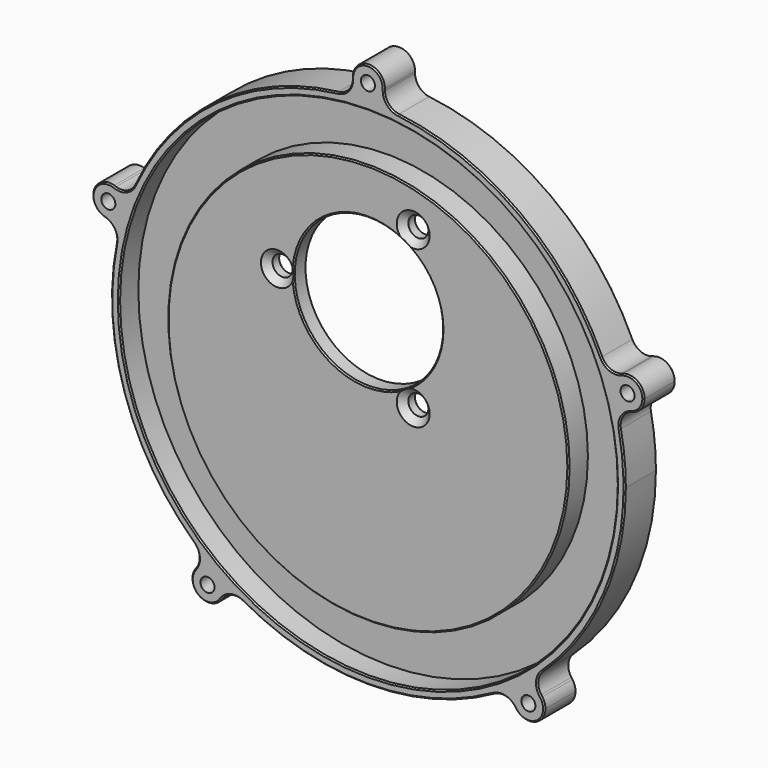
from build123d import *

# Parameters (mm, degrees)
F0_R          = 2.778125
F0_R_2        = 98.425
F1_DEPTH      = 15.875
F0_R_3        = 79.375
F0_R_4        = 3.96875
F0_R_5        = 29.36875
F2_DEPTH      = 6.35
F3_R          = 76.2
F3_R_2        = 3.96875
F3_R_3        = 29.36875
F4_DEPTH      = 9.525
F5_R          = 6.35
F7_T1_DEPTH   = 0.7496618475
F7_T3_DEPTH   = 0.7496618475
F7_T5_DEPTH   = 0.7496618475
F7_T7_DEPTH   = 0.7496618475
F7_T9_DEPTH   = 0.7496618475
F7_T11_DEPTH  = 0.7496618475
F7_T13_DEPTH  = 0.7496618475
F7_T15_DEPTH  = 0.7496618475
F7_T17_DEPTH  = 0.7496618475
F7_T20_ANGLE  = 58.4873459388
F7_T26_ANGLE  = 60.8393567081
F7_T28_ANGLE  = 121.6812910479
F7_T30_ANGLE  = 121.6812910479
F7_T32_ANGLE  = 60.8393567081
F7_T38_ANGLE  = 58.4873459388
F7_T46_ANGLE  = 83.2436729694
F7_T48_ANGLE  = 83.2436729694
F7_T50_ANGLE  = 180
F7_T52_ANGLE  = 83.2436729694
F7_T54_ANGLE  = 58.4873459388
F7_T56_ANGLE  = 83.2436729694
F7_T58_ANGLE  = 180
F7_T60_ANGLE  = 83.2436729694
F7_T62_ANGLE  = 58.4873459388
F7_T64_ANGLE  = 83.2436729694
F7_T66_ANGLE  = 180
F7_T68_ANGLE  = 83.2436729694
F7_T70_ANGLE  = 58.4873459388
F7_T72_ANGLE  = 83.2436729694
F7_T74_ANGLE  = 180
F7_T76_ANGLE  = 83.2436729694
F7_T78_ANGLE  = 58.4873459388
F7_T80_ANGLE  = 83.2436729694
F7_T82_ANGLE  = 180
F7_T84_ANGLE  = 83.2436729694
F7_T86_ANGLE  = 83.2436729694
F7_T88_ANGLE  = 180
F7_T90_ANGLE  = 83.2436729694
F7_T92_ANGLE  = 58.4873459388
F7_T94_ANGLE  = 83.2436729694
F7_T96_ANGLE  = 180
F7_T98_ANGLE  = 83.2436729694
F7_T100_ANGLE = 58.4873459388
F7_T102_ANGLE = 83.2436729694
F7_T104_ANGLE = 180
F7_T106_ANGLE = 83.2436729694
F7_T108_ANGLE = 58.4873459388
F7_T110_ANGLE = 83.2436729694
F7_T112_ANGLE = 180
F7_T114_ANGLE = 83.2436729694
F7_T116_ANGLE = 58.4873459388
F7_T118_ANGLE = 83.2436729694
F7_T120_ANGLE = 180


# Not quite as in the source:
# - a fillet or chamfer that OpenCascade refuses, or shapes differently, is made with other operations: its cross-section is extruded or revolved along the edge and cut away or added


with BuildPart() as f1:
    # F0 (on Front) → F1 (new body)
    with BuildSketch(Plane.XZ):
        with BuildLine():
            Line((-58.3141600707, -91.0658208948), (-54.4649709547, -85.7678665871))
            ThreePointArc((-54.4649709547, -85.7678665871), (-57.1199008944, -84.0230737465), (-59.7189814526, -82.1961267595))
            ThreePointArc((-59.7189814526, -82.1961267595), (-57.7935265058, -84.4505449687), (-57.101417985, -87.3333845428))
            ThreePointArc((-57.101417985, -87.3333845428), (-57.4122091065, -89.2956424571), (-58.3141600707, -91.0658208948))
        make_face()
        with BuildLine():
            ThreePointArc((-68.5886758993, -83.6009481907), (-64.4447767279, -81.0615635626), (-59.7189814526, -82.1961267595))
            ThreePointArc((-59.7189814526, -82.1961267595), (-62.2596715362, -80.2888117996), (-64.7394867833, -78.302993883))
            Line((-64.7394867833, -78.302993883), (-68.5886758993, -83.6009481907))
        make_face()
        with BuildLine():
            ThreePointArc((-57.101417985, -87.3333845428), (-57.7935265058, -84.4505449687), (-59.7189814526, -82.1961267595))
            ThreePointArc((-59.7189814526, -82.1961267595), (-64.4447767279, -81.0615635626), (-68.5886758993, -83.6009481907))
            ThreePointArc((-68.5886758993, -83.6009481907), (-67.183854337, -92.4706424571), (-58.3141600707, -91.0658208948))
            ThreePointArc((-58.3141600707, -91.0658208948), (-57.4122091065, -89.2956424571), (-57.101417985, -87.3333845428))
        make_face()
        with Locations((-63.451417985, -87.3333845428)):
            Circle(F0_R, mode=Mode.SUBTRACT)
        with BuildLine():
            Line((68.5886758993, -83.6009481907), (64.7394867833, -78.302993883))
            ThreePointArc((64.7394867833, -78.302993883), (62.2596715502, -80.2888117888), (59.7189814811, -82.1961267388))
            ThreePointArc((59.7189814811, -82.1961267388), (64.4447767453, -81.0615635653), (68.5886758993, -83.6009481907))
        make_face()
        with BuildLine():
            ThreePointArc((58.3141600707, -91.0658208948), (57.1795970075, -86.3400257824), (59.7189814811, -82.1961267388))
            ThreePointArc((59.7189814811, -82.1961267388), (57.119900909, -84.0230737366), (54.4649709547, -85.7678665871))
            Line((54.4649709547, -85.7678665871), (58.3141600707, -91.0658208948))
        make_face()
        with BuildLine():
            ThreePointArc((68.5886758993, -83.6009481907), (64.4447767453, -81.0615635653), (59.7189814811, -82.1961267388))
            ThreePointArc((59.7189814811, -82.1961267388), (57.1795970075, -86.3400257824), (58.3141600707, -91.0658208948))
            ThreePointArc((58.3141600707, -91.0658208948), (65.4136758993, -93.3725934212), (69.801417985, -87.3333845428))
            ThreePointArc((69.801417985, -87.3333845428), (69.4906268634, -85.3711266285), (68.5886758993, -83.6009481907))
        make_face()
        with Locations((63.451417985, -87.3333845428)):
            Circle(F0_R, mode=Mode.SUBTRACT)
        with BuildLine():
            ThreePointArc((94.476174201, 37.3739549465), (95.5984941663, 34.4018591524), (96.6273420327, 31.3961266988))
            ThreePointArc((96.6273420327, 31.3961266988), (97.0086595223, 36.2412242491), (100.7042930198, 39.3975934212))
            Line((100.7042930198, 39.3975934212), (94.476174201, 37.3739549465))
        make_face()
        with BuildLine():
            ThreePointArc((96.6273420327, 31.3961266988), (97.5617118577, 28.359696391), (98.4006900295, 25.2955371896))
            Line((98.4006900295, 25.2955371896), (104.6288088483, 27.3191756643))
            ThreePointArc((104.6288088483, 27.3191756643), (99.7837112278, 27.700493131), (96.6273420327, 31.3961266988))
        make_face()
        with BuildLine():
            ThreePointArc((100.7042930198, 39.3975934212), (97.0086595223, 36.2412242491), (96.6273420327, 31.3961266988))
            ThreePointArc((96.6273420327, 31.3961266988), (99.7837112278, 27.700493131), (104.6288088483, 27.3191756643))
            ThreePointArc((104.6288088483, 27.3191756643), (107.8038088483, 29.6259481907), (109.0165509341, 33.3583845428))
            ThreePointArc((109.0165509341, 33.3583845428), (106.3989872861, 38.4956424571), (100.7042930198, 39.3975934212))
        make_face()
        with Locations((102.6665509341, 33.3583845428)):
            Circle(F0_R, mode=Mode.SUBTRACT)
        with BuildLine():
            ThreePointArc((-1.426e-07, 101.6), (3.1765528772, 101.5503299444), (6.35, 101.401368334))
            Line((6.35, 101.401368334), (6.35, 107.95))
            ThreePointArc((6.35, 107.95), (4.4901280101, 103.459871889), (-1.426e-07, 101.6))
        make_face()
        with BuildLine():
            ThreePointArc((-6.35, 101.401368334), (-3.1765530198, 101.5503299399), (-1.426e-07, 101.6))
            ThreePointArc((-1.426e-07, 101.6), (-4.490128111, 103.4598719899), (-6.35, 107.95))
            Line((-6.35, 107.95), (-6.35, 101.401368334))
        make_face()
        with BuildLine():
            ThreePointArc((-6.35, 107.95), (-4.490128111, 103.4598719899), (-1.426e-07, 101.6))
            ThreePointArc((-1.426e-07, 101.6), (4.4901280101, 103.459871889), (6.35, 107.95))
            ThreePointArc((6.35, 107.95), (0, 114.3), (-6.35, 107.95))
        make_face()
        with Locations((0, 107.95)):
            Circle(F0_R, mode=Mode.SUBTRACT)
        with BuildLine():
            ThreePointArc((-96.6273420365, 31.3961266873), (-95.5984941683, 34.4018591467), (-94.476174201, 37.3739549465))
            Line((-94.476174201, 37.3739549465), (-100.7042930198, 39.3975934212))
            ThreePointArc((-100.7042930198, 39.3975934212), (-97.5292930198, 37.0908208948), (-96.3165509341, 33.3583845428))
            ThreePointArc((-96.3165509341, 33.3583845428), (-96.3947299664, 32.3650257203), (-96.6273420365, 31.3961266873))
        make_face()
        with BuildLine():
            Line((-104.6288088483, 27.3191756643), (-98.4006900295, 25.2955371896))
            ThreePointArc((-98.4006900295, 25.2955371896), (-97.5617118594, 28.3596963852), (-96.6273420365, 31.3961266873))
            ThreePointArc((-96.6273420365, 31.3961266873), (-99.7837112331, 27.7004931282), (-104.6288088483, 27.3191756643))
        make_face()
        with BuildLine():
            ThreePointArc((-104.6288088483, 27.3191756643), (-99.7837112331, 27.7004931282), (-96.6273420365, 31.3961266873))
            ThreePointArc((-96.6273420365, 31.3961266873), (-96.3947299664, 32.3650257203), (-96.3165509341, 33.3583845428))
            ThreePointArc((-96.3165509341, 33.3583845428), (-97.5292930198, 37.0908208948), (-100.7042930198, 39.3975934212))
            ThreePointArc((-100.7042930198, 39.3975934212), (-108.7057598125, 35.3206424571), (-104.6288088483, 27.3191756643))
        make_face()
        with Locations((-102.6665509341, 33.3583845428)):
            Circle(F0_R, mode=Mode.SUBTRACT)
        with BuildLine():
            ThreePointArc((64.7394867833, -78.302993883), (91.9241313725, -43.2725556376), (101.6, 0))
            ThreePointArc((101.6, 0), (100.7969992287, 12.7485272286), (98.4006900295, 25.2955371896))
            ThreePointArc((98.4006900295, 25.2955371896), (97.5617118577, 28.359696391), (96.6273420327, 31.3961266988))
            ThreePointArc((96.6273420327, 31.3961266988), (95.5984941663, 34.4018591524), (94.476174201, 37.3739549465))
            ThreePointArc((94.476174201, 37.3739549465), (59.7189816329, 82.1961266285), (6.35, 101.401368334))
            ThreePointArc((6.35, 101.401368334), (3.1765528772, 101.5503299444), (-1.426e-07, 101.6))
            ThreePointArc((-1.426e-07, 101.6), (-3.1765530198, 101.5503299399), (-6.35, 101.401368334))
            ThreePointArc((-6.35, 101.401368334), (-59.7189816329, 82.1961266285), (-94.476174201, 37.3739549465))
            ThreePointArc((-94.476174201, 37.3739549465), (-95.5984941683, 34.4018591467), (-96.6273420365, 31.3961266873))
            ThreePointArc((-96.6273420365, 31.3961266873), (-97.5617118594, 28.3596963852), (-98.4006900295, 25.2955371896))
            ThreePointArc((-98.4006900295, 25.2955371896), (-96.6273420556, -31.3961266285), (-64.7394867833, -78.302993883))
            ThreePointArc((-64.7394867833, -78.302993883), (-62.2596715362, -80.2888117996), (-59.7189814526, -82.1961267595))
            ThreePointArc((-59.7189814526, -82.1961267595), (-57.1199008944, -84.0230737465), (-54.4649709547, -85.7678665871))
            ThreePointArc((-54.4649709547, -85.7678665871), (0, -101.6), (54.4649709547, -85.7678665871))
            ThreePointArc((54.4649709547, -85.7678665871), (57.119900909, -84.0230737366), (59.7189814811, -82.1961267388))
            ThreePointArc((59.7189814811, -82.1961267388), (62.2596715502, -80.2888117888), (64.7394867833, -78.302993883))
        make_face()
        Circle(F0_R_2, mode=Mode.SUBTRACT)
    extrude(amount=F1_DEPTH)



with BuildPart() as f1b:
    # F0 (on Front) → F1, piece 2 (new body)
    with BuildSketch(Plane.XZ):
        Circle(F0_R_3)
        with Locations((17.9025847465, 0.7418136323)):
            Circle(F0_R_4, mode=Mode.SUBTRACT)
        with Locations((-35.805169493, 31.75)):
            Circle(F0_R_4, mode=Mode.SUBTRACT)
        with Locations((0, 31.75)):
            Circle(F0_R_5, mode=Mode.SUBTRACT)
        with Locations((17.9025847465, 62.7581863677)):
            Circle(F0_R_4, mode=Mode.SUBTRACT)
    extrude(amount=F1_DEPTH)


with BuildPart() as f1_1:
    add(f1.part)

    add(f1b.part)  # F2 merges F1b
    # F0 (on Front) → F2 (join)
    with BuildSketch(Plane.XZ):
        Circle(F0_R_2)
        Circle(F0_R_3, mode=Mode.SUBTRACT)
    extrude(amount=F2_DEPTH)

    # F3 (on face) → F4 (cut)
    with BuildSketch(Plane.XZ):
        Circle(F3_R)
        with Locations((-35.805169493, 31.75)):
            Circle(F3_R_2, mode=Mode.SUBTRACT)
        with Locations((17.9025847465, 0.7418136323)):
            Circle(F3_R_2, mode=Mode.SUBTRACT)
        with Locations((0, 31.75)):
            Circle(F3_R_3, mode=Mode.SUBTRACT)
        with Locations((17.9025847465, 62.7581863677)):
            Circle(F3_R_2, mode=Mode.SUBTRACT)
    extrude(amount=F4_DEPTH, mode=Mode.SUBTRACT)

    # F5
    f5_edges = [f1_1.edges().sort_by_distance(p)[0] for p in [
        (6.35, -7.9375, 101.401368),
        (94.476174, -7.9375, 37.373955),
        (64.739487, -7.9375, -78.302994),
        (54.464971, -7.9375, -85.767867),
        (-54.464971, -7.9375, -85.767867),
        (-64.739487, -7.9375, -78.302994),
        (-98.40069, -7.9375, 25.295537),
        (-94.476174, -7.9375, 37.373955),
        (-6.35, -7.9375, 101.401368),
        (98.40069, -7.9375, 25.295537),
    ]]
    fillet(f5_edges, radius=F5_R)

    # F6: chamfer of 2.54 on 3 edges, made by hand

    # F6_s1 → F6_t2 (revolve, cut)
    with BuildSketch(Plane.XY.offset(62.7581863677)):
        Polygon((24.4113347465, -15.875), (21.8713347465, -13.335), (21.8713347465, -15.875), align=None)
    revolve(axis=Axis((17.9025847465, -15.875, 62.7581863677), (0, -1, 0)), mode=Mode.SUBTRACT)

    # F6_s3 → F6_t4 (revolve, cut)
    with BuildSketch(Plane.XY.offset(0.7418136323)):
        Polygon((24.4113347465, -15.875), (21.8713347465, -13.335), (21.8713347465, -15.875), align=None)
    revolve(axis=Axis((17.9025847465, -15.875, 0.7418136323), (0, -1, 0)), mode=Mode.SUBTRACT)

    # F6_s5 → F6_t6 (revolve, cut)
    with BuildSketch(Plane.XY.offset(31.75)):
        Polygon((-29.296419493, -15.875), (-31.836419493, -13.335), (-31.836419493, -15.875), align=None)
    revolve(axis=Axis((-35.805169493, -15.875, 31.75), (0, -1, 0)), mode=Mode.SUBTRACT)

    # F7: chamfer of 0.508 on 13 edges, made by hand

    # F7_s2 → F7_t1 (cut)
    with BuildSketch(Plane(origin=(-101.9535801489, 0, 33.1267262918), x_dir=(0, 1, 0), z_dir=(-0.9510565163, 0, 0.3090169944))):
        Polygon((-0.508, -6.35), (0, -5.842), (0, -6.35), align=None)
        Polygon((-15.875, -5.842), (-15.367, -6.35), (-15.875, -6.35), align=None)
    extrude(amount=F7_T1_DEPTH, mode=Mode.SUBTRACT)

    # F7_s4 → F7_t3 (cut)
    with BuildSketch(Plane(origin=(-102.6665509341, 0, 33.3583845428), x_dir=(0, 1, 0), z_dir=(0.9510565163, 0, -0.3090169944))):
        Polygon((-0.508, -6.35), (0, -5.842), (0, -6.35), align=None)
        Polygon((-15.875, -5.842), (-15.367, -6.35), (-15.875, -6.35), align=None)
    extrude(amount=F7_T3_DEPTH, mode=Mode.SUBTRACT)

    # F7_s6 → F7_t5 (cut)
    with BuildSketch(Plane(origin=(-63.0107778068, 0, -86.7268953681), x_dir=(0, 1, 0), z_dir=(-0.5877852523, 0, -0.8090169944))):
        Polygon((-0.508, -6.35), (0, -5.842), (0, -6.35), align=None)
        Polygon((-15.875, -5.842), (-15.367, -6.35), (-15.875, -6.35), align=None)
    extrude(amount=F7_T5_DEPTH, mode=Mode.SUBTRACT)

    # F7_s8 → F7_t7 (cut)
    with BuildSketch(Plane(origin=(-63.451417985, 0, -87.3333845428), x_dir=(0, 1, 0), z_dir=(0.5877852523, 0, 0.8090169944))):
        Polygon((-0.508, -6.35), (0, -5.842), (0, -6.35), align=None)
        Polygon((-15.875, -5.842), (-15.367, -6.35), (-15.875, -6.35), align=None)
    extrude(amount=F7_T7_DEPTH, mode=Mode.SUBTRACT)

    # F7_s10 → F7_t9 (cut)
    with BuildSketch(Plane(origin=(63.0107778068, 0, -86.7268953681), x_dir=(0, 1, 0), z_dir=(0.5877852523, 0, -0.8090169944))):
        Polygon((-0.508, -6.35), (0, -5.842), (0, -6.35), align=None)
        Polygon((-15.875, -5.842), (-15.367, -6.35), (-15.875, -6.35), align=None)
    extrude(amount=F7_T9_DEPTH, mode=Mode.SUBTRACT)

    # F7_s12 → F7_t11 (cut)
    with BuildSketch(Plane(origin=(63.451417985, 0, -87.3333845428), x_dir=(0, 1, 0), z_dir=(-0.5877852523, 0, 0.8090169944))):
        Polygon((-0.508, -6.35), (0, -5.842), (0, -6.35), align=None)
        Polygon((-15.875, -5.842), (-15.367, -6.35), (-15.875, -6.35), align=None)
    extrude(amount=F7_T11_DEPTH, mode=Mode.SUBTRACT)

    # F7_s14 → F7_t13 (cut)
    with BuildSketch(Plane(origin=(101.9535801489, 0, 33.1267262918), x_dir=(0, 1, 0), z_dir=(0.9510565163, 0, 0.3090169944))):
        Polygon((-0.508, -6.35), (0, -5.842), (0, -6.35), align=None)
        Polygon((-15.875, -5.842), (-15.367, -6.35), (-15.875, -6.35), align=None)
    extrude(amount=F7_T13_DEPTH, mode=Mode.SUBTRACT)

    # F7_s16 → F7_t15 (cut)
    with BuildSketch(Plane(origin=(102.6665509341, 0, 33.3583845428), x_dir=(0, 1, 0), z_dir=(-0.9510565163, 0, -0.3090169944))):
        Polygon((-0.508, -6.35), (0, -5.842), (0, -6.35), align=None)
        Polygon((-15.875, -5.842), (-15.367, -6.35), (-15.875, -6.35), align=None)
    extrude(amount=F7_T15_DEPTH, mode=Mode.SUBTRACT)

    # F7_s18 → F7_t17 (cut)
    with BuildSketch(Plane.XY.offset(107.2003381525)):
        Polygon((6.35, -0.508), (5.842, 0), (6.35, 0), align=None)
        Polygon((-6.35, -0.508), (-5.842, 0), (-6.35, 0), align=None)
        Polygon((5.842, -15.875), (6.35, -15.367), (6.35, -15.875), align=None)
        Polygon((-5.842, -15.875), (-6.35, -15.367), (-6.35, -15.875), align=None)
    extrude(amount=F7_T17_DEPTH, mode=Mode.SUBTRACT)

    # F7_s19 → F7_t20 (revolve, cut)
    with BuildSketch(Plane(origin=(0, 0, 0), x_dir=(0, 1, 0), z_dir=(0.418760019, 0, -0.9080969367))):
        Polygon((-15.875, 101.092), (-15.367, 101.6), (-15.875, 101.6), align=None)
    revolve(axis=Axis((0, -15.875, 0), (0, -1, 0)), revolution_arc=F7_T20_ANGLE, mode=Mode.SUBTRACT)

    # F7_s21 → F7_t22 (revolve, cut)
    with BuildSketch(Plane.XY):
        Polygon((79.375, -15.367), (78.867, -15.875), (79.375, -15.875), align=None)
    revolve(axis=Axis((0, -15.875, 0), (0, -1, 0)), mode=Mode.SUBTRACT)

    # F7_s23 → F7_t24 (revolve, cut)
    with BuildSketch(Plane.XY):
        Polygon((98.933, -15.875), (98.425, -15.367), (98.425, -15.875), align=None)
    revolve(axis=Axis((0, -15.875, 0), (0, -1, 0)), mode=Mode.SUBTRACT)

    # F7_s25 → F7_t26 (revolve, cut)
    with BuildSketch(Plane.XY.offset(31.75)):
        Polygon((29.87675, -15.875), (29.36875, -15.367), (29.36875, -15.875), align=None)
    revolve(axis=Axis((0, -15.875, 31.75), (0, -1, 0)), revolution_arc=F7_T26_ANGLE, mode=Mode.SUBTRACT)

    # F7_s27 → F7_t28 (revolve, cut)
    with BuildSketch(Plane(origin=(-13.9751197067, 0, 8.3442859446), x_dir=(0, 1, 0), z_dir=(0.8585964385, 0, -0.5126520806))):
        Polygon((-15.875, 57.1371869235), (-15.367, 56.6291869235), (-15.875, 56.6291869235), align=None)
    revolve(axis=Axis((0, -15.875, 31.75), (0, -1, 0)), revolution_arc=F7_T28_ANGLE, mode=Mode.SUBTRACT)

    # F7_s29 → F7_t30 (revolve, cut)
    with BuildSketch(Plane(origin=(0.4657701732, 0, 31.7431657146), x_dir=(0, 1, 0), z_dir=(0.0146715058, 0, 0.9998923677))):
        Polygon((-15.875, 30.3425703105), (-15.367, 29.8345703105), (-15.875, 29.8345703105), align=None)
    revolve(axis=Axis((0, -15.875, 31.75), (0, -1, 0)), revolution_arc=F7_T30_ANGLE, mode=Mode.SUBTRACT)

    # F7_s31 → F7_t32 (revolve, cut)
    with BuildSketch(Plane(origin=(13.5097246067, 0, 7.5381561098), x_dir=(0, 1, 0), z_dir=(-0.8732569841, 0, -0.4872599303))):
        Polygon((-15.875, 2.1508407541), (-15.367, 1.6428407541), (-15.875, 1.6428407541), align=None)
    revolve(axis=Axis((0, -15.875, 31.75), (0, -1, 0)), revolution_arc=F7_T32_ANGLE, mode=Mode.SUBTRACT)

    # F7_s33 → F7_t34 (revolve, cut)
    with BuildSketch(Plane.XY.offset(31.75)):
        Polygon((29.87675, -9.525), (29.36875, -10.033), (29.36875, -9.525), align=None)
    revolve(axis=Axis((0, -9.525, 31.75), (0, -1, 0)), mode=Mode.SUBTRACT)

    # F7_s35 → F7_t36 (revolve, cut)
    with BuildSketch(Plane.XY):
        Polygon((76.708, 0), (76.2, -0.508), (76.2, 0), align=None)
    revolve(axis=Axis((0, 0, 0), (0, -1, 0)), mode=Mode.SUBTRACT)

    # F7_s37 → F7_t38 (revolve, cut)
    with BuildSketch(Plane(origin=(0, 0, 0), x_dir=(0, 1, 0), z_dir=(0.9930554715, 0, 0.1176470588))):
        Polygon((-0.508, 101.6), (0, 101.092), (0, 101.6), align=None)
    revolve(axis=Axis((0, 0, 0), (0, -1, 0)), revolution_arc=F7_T38_ANGLE, mode=Mode.SUBTRACT)

    # F7_s39 → F7_t40 (revolve, cut)
    with BuildSketch(Plane.XY.offset(62.7581863677)):
        Polygon((22.3793347465, -9.525), (21.8713347465, -10.033), (21.8713347465, -9.525), align=None)
    revolve(axis=Axis((17.9025847465, -9.525, 62.7581863677), (0, -1, 0)), mode=Mode.SUBTRACT)

    # F7_s41 → F7_t42 (revolve, cut)
    with BuildSketch(Plane.XY.offset(31.75)):
        Polygon((-31.328419493, -9.525), (-31.836419493, -10.033), (-31.836419493, -9.525), align=None)
    revolve(axis=Axis((-35.805169493, -9.525, 31.75), (0, -1, 0)), mode=Mode.SUBTRACT)

    # F7_s43 → F7_t44 (revolve, cut)
    with BuildSketch(Plane.XY.offset(0.7418136323)):
        Polygon((22.3793347465, -9.525), (21.8713347465, -10.033), (21.8713347465, -9.525), align=None)
    revolve(axis=Axis((17.9025847465, -9.525, 0.7418136323), (0, -1, 0)), mode=Mode.SUBTRACT)

    # F7_s45 → F7_t46 (revolve, cut)
    with BuildSketch(Plane.XY.offset(107.2003381525)):
        Polygon((-6.35, -0.508), (-5.842, 0), (-6.35, 0), align=None)
    revolve(axis=Axis((-12.7, 0, 107.2003381525), (0, 1, 0)), revolution_arc=F7_T46_ANGLE, mode=Mode.SUBTRACT)

    # F7_s47 → F7_t48 (revolve, cut)
    with BuildSketch(Plane(origin=(0, 0, 0), x_dir=(0, 1, 0), z_dir=(0.418760019, 0, 0.9080969367))):
        Polygon((-0.508, 101.6), (0, 101.092), (0, 101.6), align=None)
    revolve(axis=Axis((-98.0290643204, 0, 45.2051440488), (0, 1, 0)), revolution_arc=F7_T48_ANGLE, mode=Mode.SUBTRACT)

    # F7_s49 → F7_t50 (revolve, cut)
    with BuildSketch(Plane(origin=(-102.6665509341, 0, 33.3583845428), x_dir=(0, 1, 0), z_dir=(0.9510565163, 0, -0.3090169944))):
        Polygon((-0.508, 6.35), (0, 5.842), (0, 6.35), align=None)
    revolve(axis=Axis((-102.6665509341, 0, 33.3583845428), (0, -1, 0)), revolution_arc=F7_T50_ANGLE, mode=Mode.SUBTRACT)

    # F7_s51 → F7_t52 (revolve, cut)
    with BuildSketch(Plane(origin=(-101.9535801489, 0, 33.1267262918), x_dir=(0, 1, 0), z_dir=(-0.9510565163, 0, 0.3090169944))):
        Polygon((-0.508, 6.35), (0, 5.842), (0, 6.35), align=None)
    revolve(axis=Axis((-105.8780959775, 0, 21.0483085349), (0, 1, 0)), revolution_arc=F7_T52_ANGLE, mode=Mode.SUBTRACT)

    # F7_s53 → F7_t54 (revolve, cut)
    with BuildSketch(Plane(origin=(0, 0, 0), x_dir=(0, 1, 0), z_dir=(0.1949820151, 0, 0.9808068178))):
        Polygon((-0.508, 101.6), (0, 101.092), (0, 101.6), align=None)
    revolve(axis=Axis((0, 0, 0), (0, -1, 0)), revolution_arc=F7_T54_ANGLE, mode=Mode.SUBTRACT)

    # F7_s55 → F7_t56 (revolve, cut)
    with BuildSketch(Plane(origin=(0, 0, 0), x_dir=(0, 1, 0), z_dir=(-0.7342475467, 0, 0.6788818308))):
        Polygon((-0.508, 101.6), (0, 101.092), (0, 101.6), align=None)
    revolve(axis=Axis((-73.2852936353, 0, -79.262022664), (0, 1, 0)), revolution_arc=F7_T56_ANGLE, mode=Mode.SUBTRACT)

    # F7_s57 → F7_t58 (revolve, cut)
    with BuildSketch(Plane(origin=(-63.451417985, 0, -87.3333845428), x_dir=(0, 1, 0), z_dir=(0.5877852523, 0, 0.8090169944))):
        Polygon((-0.508, 6.35), (0, 5.842), (0, 6.35), align=None)
    revolve(axis=Axis((-63.451417985, 0, -87.3333845428), (0, -1, 0)), revolution_arc=F7_T58_ANGLE, mode=Mode.SUBTRACT)

    # F7_s59 → F7_t60 (revolve, cut)
    with BuildSketch(Plane(origin=(-63.0107778068, 0, -86.7268953681), x_dir=(0, 1, 0), z_dir=(-0.5877852523, 0, -0.8090169944))):
        Polygon((-0.508, 6.35), (0, 5.842), (0, 6.35), align=None)
    revolve(axis=Axis((-52.7362619782, 0, -94.1917680722), (0, 1, 0)), revolution_arc=F7_T60_ANGLE, mode=Mode.SUBTRACT)

    # F7_s61 → F7_t62 (revolve, cut)
    with BuildSketch(Plane(origin=(0, 0, 0), x_dir=(0, 1, 0), z_dir=(-0.872549959, 0, 0.488524891))):
        Polygon((-0.508, 101.6), (0, 101.092), (0, 101.6), align=None)
    revolve(axis=Axis((0, 0, 0), (0, -1, 0)), revolution_arc=F7_T62_ANGLE, mode=Mode.SUBTRACT)

    # F7_s63 → F7_t64 (revolve, cut)
    with BuildSketch(Plane(origin=(0, 0, 0), x_dir=(0, 1, 0), z_dir=(-0.872549959, 0, -0.488524891))):
        Polygon((-0.508, 101.6), (0, 101.092), (0, 101.6), align=None)
    revolve(axis=Axis((52.7362619782, 0, -94.1917680722), (0, 1, 0)), revolution_arc=F7_T64_ANGLE, mode=Mode.SUBTRACT)

    # F7_s65 → F7_t66 (revolve, cut)
    with BuildSketch(Plane(origin=(63.451417985, 0, -87.3333845428), x_dir=(0, 1, 0), z_dir=(-0.5877852523, 0, 0.8090169944))):
        Polygon((-0.508, 6.35), (0, 5.842), (0, 6.35), align=None)
    revolve(axis=Axis((63.451417985, 0, -87.3333845428), (0, -1, 0)), revolution_arc=F7_T66_ANGLE, mode=Mode.SUBTRACT)

    # F7_s67 → F7_t68 (revolve, cut)
    with BuildSketch(Plane(origin=(63.0107778068, 0, -86.7268953681), x_dir=(0, 1, 0), z_dir=(0.5877852523, 0, -0.8090169944))):
        Polygon((-0.508, 6.35), (0, 5.842), (0, 6.35), align=None)
    revolve(axis=Axis((73.2852936353, 0, -79.262022664), (0, 1, 0)), revolution_arc=F7_T68_ANGLE, mode=Mode.SUBTRACT)

    # F7_s69 → F7_t70 (revolve, cut)
    with BuildSketch(Plane(origin=(0, 0, 0), x_dir=(0, 1, 0), z_dir=(-0.7342475467, 0, -0.6788818308))):
        Polygon((-0.508, 101.6), (0, 101.092), (0, 101.6), align=None)
    revolve(axis=Axis((0, 0, 0), (0, -1, 0)), revolution_arc=F7_T70_ANGLE, mode=Mode.SUBTRACT)

    # F7_s71 → F7_t72 (revolve, cut)
    with BuildSketch(Plane(origin=(0, 0, 0), x_dir=(0, 1, 0), z_dir=(0.1949820151, 0, -0.9808068178))):
        Polygon((-0.508, 101.6), (0, 101.092), (0, 101.6), align=None)
    revolve(axis=Axis((105.8780959775, 0, 21.0483085349), (0, 1, 0)), revolution_arc=F7_T72_ANGLE, mode=Mode.SUBTRACT)

    # F7_s73 → F7_t74 (revolve, cut)
    with BuildSketch(Plane(origin=(102.6665509341, 0, 33.3583845428), x_dir=(0, 1, 0), z_dir=(-0.9510565163, 0, -0.3090169944))):
        Polygon((-0.508, 6.35), (0, 5.842), (0, 6.35), align=None)
    revolve(axis=Axis((102.6665509341, 0, 33.3583845428), (0, -1, 0)), revolution_arc=F7_T74_ANGLE, mode=Mode.SUBTRACT)

    # F7_s75 → F7_t76 (revolve, cut)
    with BuildSketch(Plane(origin=(101.9535801489, 0, 33.1267262918), x_dir=(0, 1, 0), z_dir=(0.9510565163, 0, 0.3090169944))):
        Polygon((-0.508, 6.35), (0, 5.842), (0, 6.35), align=None)
    revolve(axis=Axis((98.0290643204, 0, 45.2051440488), (0, 1, 0)), revolution_arc=F7_T76_ANGLE, mode=Mode.SUBTRACT)

    # F7_s77 → F7_t78 (revolve, cut)
    with BuildSketch(Plane(origin=(0, 0, 0), x_dir=(0, 1, 0), z_dir=(0.418760019, 0, -0.9080969367))):
        Polygon((-0.508, 101.6), (0, 101.092), (0, 101.6), align=None)
    revolve(axis=Axis((0, 0, 0), (0, -1, 0)), revolution_arc=F7_T78_ANGLE, mode=Mode.SUBTRACT)

    # F7_s79 → F7_t80 (revolve, cut)
    with BuildSketch(Plane(origin=(0, 0, 0), x_dir=(0, 1, 0), z_dir=(0.9930554715, 0, -0.1176470588))):
        Polygon((-0.508, 101.6), (0, 101.092), (0, 101.6), align=None)
    revolve(axis=Axis((12.7, 0, 107.2003381525), (0, 1, 0)), revolution_arc=F7_T80_ANGLE, mode=Mode.SUBTRACT)

    # F7_s81 → F7_t82 (revolve, cut)
    with BuildSketch(Plane.XY.offset(107.95)):
        Polygon((6.35, -0.508), (5.842, 0), (6.35, 0), align=None)
    revolve(axis=Axis((0, 0, 107.95), (0, -1, 0)), revolution_arc=F7_T82_ANGLE, mode=Mode.SUBTRACT)

    # F7_s83 → F7_t84 (revolve, cut)
    with BuildSketch(Plane(origin=(101.9535801489, 0, 33.1267262918), x_dir=(0, 1, 0), z_dir=(0.9510565163, 0, 0.3090169944))):
        Polygon((-15.875, 5.842), (-15.367, 6.35), (-15.875, 6.35), align=None)
    revolve(axis=Axis((98.0290643204, -15.875, 45.2051440488), (0, 1, 0)), revolution_arc=F7_T84_ANGLE, mode=Mode.SUBTRACT)

    # F7_s85 → F7_t86 (revolve, cut)
    with BuildSketch(Plane(origin=(0, 0, 0), x_dir=(0, 1, 0), z_dir=(0.9930554715, 0, -0.1176470588))):
        Polygon((-15.875, 101.092), (-15.367, 101.6), (-15.875, 101.6), align=None)
    revolve(axis=Axis((12.7, -15.875, 107.2003381525), (0, 1, 0)), revolution_arc=F7_T86_ANGLE, mode=Mode.SUBTRACT)

    # F7_s87 → F7_t88 (revolve, cut)
    with BuildSketch(Plane.XY.offset(107.95)):
        Polygon((5.842, -15.875), (6.35, -15.367), (6.35, -15.875), align=None)
    revolve(axis=Axis((0, -15.875, 107.95), (0, -1, 0)), revolution_arc=F7_T88_ANGLE, mode=Mode.SUBTRACT)

    # F7_s89 → F7_t90 (revolve, cut)
    with BuildSketch(Plane.XY.offset(107.2003381525)):
        Polygon((-5.842, -15.875), (-6.35, -15.367), (-6.35, -15.875), align=None)
    revolve(axis=Axis((-12.7, -15.875, 107.2003381525), (0, 1, 0)), revolution_arc=F7_T90_ANGLE, mode=Mode.SUBTRACT)

    # F7_s91 → F7_t92 (revolve, cut)
    with BuildSketch(Plane(origin=(0, 0, 0), x_dir=(0, 1, 0), z_dir=(0.9930554715, 0, 0.1176470588))):
        Polygon((-15.875, 101.092), (-15.367, 101.6), (-15.875, 101.6), align=None)
    revolve(axis=Axis((0, -15.875, 0), (0, -1, 0)), revolution_arc=F7_T92_ANGLE, mode=Mode.SUBTRACT)

    # F7_s93 → F7_t94 (revolve, cut)
    with BuildSketch(Plane(origin=(0, 0, 0), x_dir=(0, 1, 0), z_dir=(0.418760019, 0, 0.9080969367))):
        Polygon((-15.875, 101.092), (-15.367, 101.6), (-15.875, 101.6), align=None)
    revolve(axis=Axis((-98.0290643204, -15.875, 45.2051440488), (0, 1, 0)), revolution_arc=F7_T94_ANGLE, mode=Mode.SUBTRACT)

    # F7_s95 → F7_t96 (revolve, cut)
    with BuildSketch(Plane(origin=(-102.6665509341, 0, 33.3583845428), x_dir=(0, 1, 0), z_dir=(0.9510565163, 0, -0.3090169944))):
        Polygon((-15.875, 5.842), (-15.367, 6.35), (-15.875, 6.35), align=None)
    revolve(axis=Axis((-102.6665509341, -15.875, 33.3583845428), (0, -1, 0)), revolution_arc=F7_T96_ANGLE, mode=Mode.SUBTRACT)

    # F7_s97 → F7_t98 (revolve, cut)
    with BuildSketch(Plane(origin=(-101.9535801489, 0, 33.1267262918), x_dir=(0, 1, 0), z_dir=(-0.9510565163, 0, 0.3090169944))):
        Polygon((-15.875, 5.842), (-15.367, 6.35), (-15.875, 6.35), align=None)
    revolve(axis=Axis((-105.8780959775, -15.875, 21.0483085349), (0, 1, 0)), revolution_arc=F7_T98_ANGLE, mode=Mode.SUBTRACT)

    # F7_s99 → F7_t100 (revolve, cut)
    with BuildSketch(Plane(origin=(0, 0, 0), x_dir=(0, 1, 0), z_dir=(0.1949820151, 0, 0.9808068178))):
        Polygon((-15.875, 101.092), (-15.367, 101.6), (-15.875, 101.6), align=None)
    revolve(axis=Axis((0, -15.875, 0), (0, -1, 0)), revolution_arc=F7_T100_ANGLE, mode=Mode.SUBTRACT)

    # F7_s101 → F7_t102 (revolve, cut)
    with BuildSketch(Plane(origin=(0, 0, 0), x_dir=(0, 1, 0), z_dir=(-0.7342475467, 0, 0.6788818308))):
        Polygon((-15.875, 101.092), (-15.367, 101.6), (-15.875, 101.6), align=None)
    revolve(axis=Axis((-73.2852936353, -15.875, -79.262022664), (0, 1, 0)), revolution_arc=F7_T102_ANGLE, mode=Mode.SUBTRACT)

    # F7_s103 → F7_t104 (revolve, cut)
    with BuildSketch(Plane(origin=(-63.451417985, 0, -87.3333845428), x_dir=(0, 1, 0), z_dir=(0.5877852523, 0, 0.8090169944))):
        Polygon((-15.875, 5.842), (-15.367, 6.35), (-15.875, 6.35), align=None)
    revolve(axis=Axis((-63.451417985, -15.875, -87.3333845428), (0, -1, 0)), revolution_arc=F7_T104_ANGLE, mode=Mode.SUBTRACT)

    # F7_s105 → F7_t106 (revolve, cut)
    with BuildSketch(Plane(origin=(-63.0107778068, 0, -86.7268953681), x_dir=(0, 1, 0), z_dir=(-0.5877852523, 0, -0.8090169944))):
        Polygon((-15.875, 5.842), (-15.367, 6.35), (-15.875, 6.35), align=None)
    revolve(axis=Axis((-52.7362619782, -15.875, -94.1917680722), (0, 1, 0)), revolution_arc=F7_T106_ANGLE, mode=Mode.SUBTRACT)

    # F7_s107 → F7_t108 (revolve, cut)
    with BuildSketch(Plane(origin=(0, 0, 0), x_dir=(0, 1, 0), z_dir=(-0.872549959, 0, 0.488524891))):
        Polygon((-15.875, 101.092), (-15.367, 101.6), (-15.875, 101.6), align=None)
    revolve(axis=Axis((0, -15.875, 0), (0, -1, 0)), revolution_arc=F7_T108_ANGLE, mode=Mode.SUBTRACT)

    # F7_s109 → F7_t110 (revolve, cut)
    with BuildSketch(Plane(origin=(0, 0, 0), x_dir=(0, 1, 0), z_dir=(-0.872549959, 0, -0.488524891))):
        Polygon((-15.875, 101.092), (-15.367, 101.6), (-15.875, 101.6), align=None)
    revolve(axis=Axis((52.7362619782, -15.875, -94.1917680722), (0, 1, 0)), revolution_arc=F7_T110_ANGLE, mode=Mode.SUBTRACT)

    # F7_s111 → F7_t112 (revolve, cut)
    with BuildSketch(Plane(origin=(63.451417985, 0, -87.3333845428), x_dir=(0, 1, 0), z_dir=(-0.5877852523, 0, 0.8090169944))):
        Polygon((-15.875, 5.842), (-15.367, 6.35), (-15.875, 6.35), align=None)
    revolve(axis=Axis((63.451417985, -15.875, -87.3333845428), (0, -1, 0)), revolution_arc=F7_T112_ANGLE, mode=Mode.SUBTRACT)

    # F7_s113 → F7_t114 (revolve, cut)
    with BuildSketch(Plane(origin=(63.0107778068, 0, -86.7268953681), x_dir=(0, 1, 0), z_dir=(0.5877852523, 0, -0.8090169944))):
        Polygon((-15.875, 5.842), (-15.367, 6.35), (-15.875, 6.35), align=None)
    revolve(axis=Axis((73.2852936353, -15.875, -79.262022664), (0, 1, 0)), revolution_arc=F7_T114_ANGLE, mode=Mode.SUBTRACT)

    # F7_s115 → F7_t116 (revolve, cut)
    with BuildSketch(Plane(origin=(0, 0, 0), x_dir=(0, 1, 0), z_dir=(-0.7342475467, 0, -0.6788818308))):
        Polygon((-15.875, 101.092), (-15.367, 101.6), (-15.875, 101.6), align=None)
    revolve(axis=Axis((0, -15.875, 0), (0, -1, 0)), revolution_arc=F7_T116_ANGLE, mode=Mode.SUBTRACT)

    # F7_s117 → F7_t118 (revolve, cut)
    with BuildSketch(Plane(origin=(0, 0, 0), x_dir=(0, 1, 0), z_dir=(0.1949820151, 0, -0.9808068178))):
        Polygon((-15.875, 101.092), (-15.367, 101.6), (-15.875, 101.6), align=None)
    revolve(axis=Axis((105.8780959775, -15.875, 21.0483085349), (0, 1, 0)), revolution_arc=F7_T118_ANGLE, mode=Mode.SUBTRACT)

    # F7_s119 → F7_t120 (revolve, cut)
    with BuildSketch(Plane(origin=(102.6665509341, 0, 33.3583845428), x_dir=(0, 1, 0), z_dir=(-0.9510565163, 0, -0.3090169944))):
        Polygon((-15.875, 5.842), (-15.367, 6.35), (-15.875, 6.35), align=None)
    revolve(axis=Axis((102.6665509341, -15.875, 33.3583845428), (0, -1, 0)), revolution_arc=F7_T120_ANGLE, mode=Mode.SUBTRACT)


solid = f1_1.part
